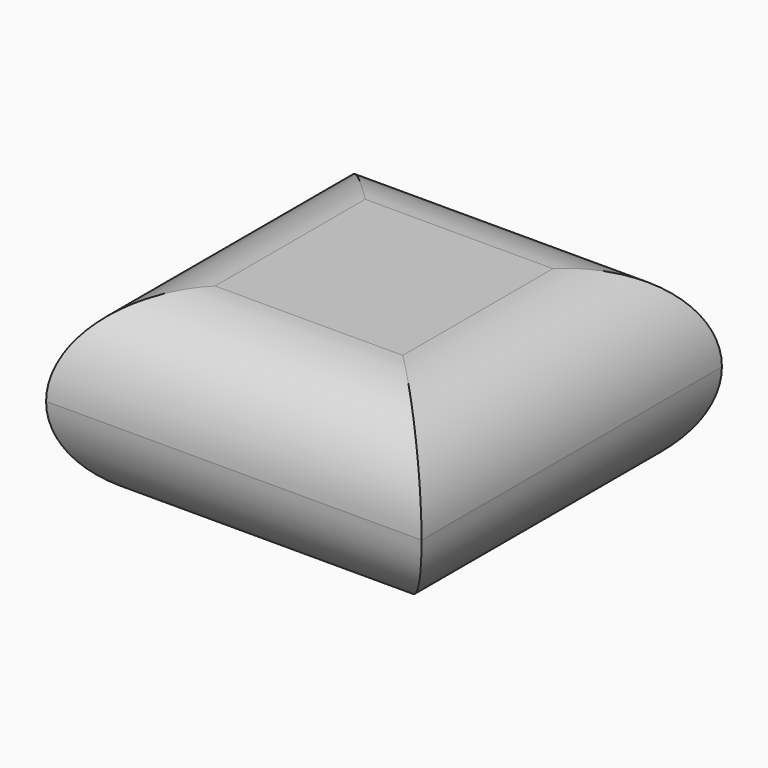
from build123d import *

# Parameters (mm, degrees)
F0_W     = 203.2
F0_H     = 203.2
F1_DEPTH = 101.6
F2_R     = 50.79999


# Not quite as in the source:
# - a fillet or chamfer is up to 0.001 mm smaller than in the source, because OpenCascade refuses the exact size


with BuildPart() as f1:
    # F0 (on Top) → F1 (new body)
    with BuildSketch(Plane.XY):
        Rectangle(F0_W, F0_H)
    extrude(amount=F1_DEPTH)

    # F2 (radius 50.8 in the source; OpenCascade refuses exactly that, so slightly less here)
    f2_edges = [f1.edges().sort_by_distance(p)[0] for p in [
        (-101.6, 0, 101.6),
        (-101.6, 0, 0),
        (101.6, 0, 0),
        (101.6, 0, 101.6),
        (0, -101.6, 101.6),
        (0, -101.6, 0),
        (0, 101.6, 101.6),
        (0, 101.6, 0),
    ]]
    fillet(f2_edges, radius=F2_R)


solid = f1.part
